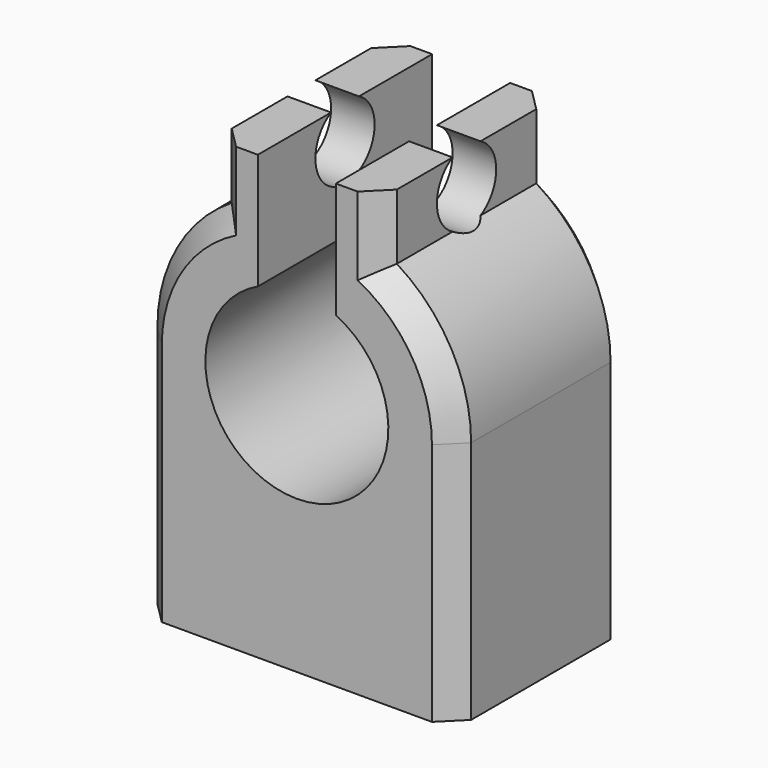
from build123d import *

# Parameters (mm, degrees)
F1_DEPTH = 10
F3_DEPTH = 4
F4_DEPTH = 20
F5_R     = 1.2
F6_DEPTH = 6
F7_SIZE  = 1


with BuildPart() as f1:
    # F0 (on Front) → F1 (new body)
    with BuildSketch(Plane.XZ):
        with BuildLine():
            ThreePointArc((1.7895, 3.7996960076), (0, -4.2), (-1.7895, 3.7996960076))
            Line((-1.7895, 3.7996960076), (-1.7895, 6.9740726803))
            Line((-1.7895, 6.9740726803), (-1.7895, 9.1220658074))
            Line((-1.7895, 9.1220658074), (-3.7895, 9.1220658074))
            Line((-3.7895, 9.1220658074), (-3.7895, 6.1220658074))
            ThreePointArc((-3.7895, 6.1220658074), (-6.2898489648, 3.5039691779), (-7.2, 0))
            Line((-7.2, 0), (-7.2, -11.2))
            Line((-7.2, -11.2), (7.2, -11.2))
            Line((7.2, -11.2), (7.2, 0))
            ThreePointArc((7.2, 0), (6.2898489648, 3.5039691779), (3.7895, 6.1220658074))
            Line((3.7895, 6.1220658074), (3.7895, 9.1220658074))
            Line((3.7895, 9.1220658074), (1.7895, 9.1220658074))
            Line((1.7895, 9.1220658074), (1.7895, 6.9740726803))
            Line((1.7895, 6.9740726803), (1.7895, 3.7996960076))
        make_face()
    extrude(amount=F1_DEPTH)

    # F2 (on face) → F3 (cut)
    with BuildSketch(Plane(origin=(-3.7895, 0, 0), x_dir=(0, -1, 0), z_dir=(-1, 0, 0))):
        with BuildLine():
            ThreePointArc((5.8, 9.1220658074), (6.4577379737, 8.4967085916), (6.7, 7.6220658074))
            ThreePointArc((6.7, 7.6220658074), (6.4577379737, 6.7474230232), (5.8, 6.1220658074))
            Line((5.8, 6.1220658074), (8.1622776602, 6.1220658074))
            ThreePointArc((8.1622776602, 6.1220658074), (8.4145257219, 6.8532913966), (8.5, 7.6220658074))
            ThreePointArc((8.5, 7.6220658074), (8.4145257219, 8.3908402182), (8.1622776602, 9.1220658074))
            Line((8.1622776602, 9.1220658074), (5.8, 9.1220658074))
        make_face()
        with BuildLine():
            ThreePointArc((4.2, 9.1220658074), (5, 9.3220658074), (5.8, 9.1220658074))
            Line((5.8, 9.1220658074), (8.1622776602, 9.1220658074))
            ThreePointArc((8.1622776602, 9.1220658074), (5, 11.1220658074), (1.8377223398, 9.1220658074))
            Line((1.8377223398, 9.1220658074), (4.2, 9.1220658074))
        make_face()
        with BuildLine():
            Line((8.1622776602, 6.1220658074), (5.8, 6.1220658074))
            ThreePointArc((5.8, 6.1220658074), (5, 5.9220658074), (4.2, 6.1220658074))
            Line((4.2, 6.1220658074), (1.8377223398, 6.1220658074))
            ThreePointArc((1.8377223398, 6.1220658074), (5, 4.1220658074), (8.1622776602, 6.1220658074))
        make_face()
        with BuildLine():
            ThreePointArc((4.2, 6.1220658074), (3.3, 7.6220658074), (4.2, 9.1220658074))
            Line((4.2, 9.1220658074), (1.8377223398, 9.1220658074))
            ThreePointArc((1.8377223398, 9.1220658074), (1.5, 7.6220658074), (1.8377223398, 6.1220658074))
            Line((1.8377223398, 6.1220658074), (4.2, 6.1220658074))
        make_face()
    extrude(amount=F3_DEPTH, mode=Mode.SUBTRACT)

    # F2 (on face) → F4 (cut, symmetric)
    with BuildSketch(Plane(origin=(-3.7895, 0, 0), x_dir=(0, -1, 0), z_dir=(-1, 0, 0))):
        with BuildLine():
            Line((4.2, 9.1220658074), (5.8, 9.1220658074))
            ThreePointArc((5.8, 9.1220658074), (5, 9.3220658074), (4.2, 9.1220658074))
        make_face()
        with BuildLine():
            ThreePointArc((5.8, 6.1220658074), (6.4577379737, 6.7474230232), (6.7, 7.6220658074))
            ThreePointArc((6.7, 7.6220658074), (6.4577379737, 8.4967085916), (5.8, 9.1220658074))
            Line((5.8, 9.1220658074), (4.2, 9.1220658074))
            ThreePointArc((4.2, 9.1220658074), (3.3, 7.6220658074), (4.2, 6.1220658074))
            Line((4.2, 6.1220658074), (5.8, 6.1220658074))
        make_face()
        with BuildLine():
            ThreePointArc((4.2, 6.1220658074), (5, 5.9220658074), (5.8, 6.1220658074))
            Line((5.8, 6.1220658074), (4.2, 6.1220658074))
        make_face()
    extrude(amount=F4_DEPTH, both=True, mode=Mode.SUBTRACT)

    # F5 (on face) → F6 (cut)
    with BuildSketch(Plane(origin=(0, 0, -11.2), x_dir=(1, 0, 0), z_dir=(0, 0, -1))):
        with Locations((-5, 3.5)):
            Circle(F5_R)
        with Locations((5, 3.5)):
            Circle(F5_R)
    extrude(amount=-F6_DEPTH, mode=Mode.SUBTRACT)

    # F7
    f7_edges = [f1.edges().sort_by_distance(p)[0] for p in [
        (7.2, 0, -5.6),
        (7.2, -10, -5.6),
        (-7.2, -10, -5.6),
        (-7.2, 0, -5.6),
        (3.7895, -10, 7.622066),
        (3.7895, 0, 7.622066),
        (-3.7895, -10, 7.622066),
        (-3.7895, 0, 7.622066),
        (-6.289849, 0, 3.503969),
        (6.289849, 0, 3.503969),
        (-6.289849, -10, 3.503969),
        (6.289849, -10, 3.503969),
    ]]
    chamfer(f7_edges, length=F7_SIZE)


solid = f1.part
